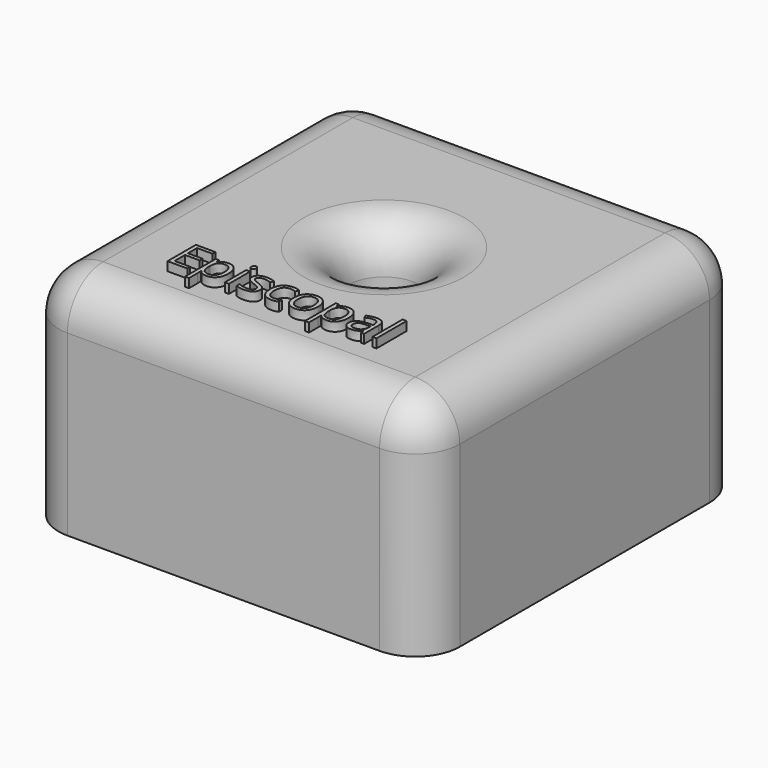
from build123d import *

# Parameters (mm, degrees)
F0_W         = 45
F0_H         = 45
F1_DEPTH     = 25
F2_R         = 4
F3_DEPTH     = 20
F4_R         = 5
F5_TEXT_SIZE = 5.5555555556
F6_DEPTH     = 1


# Not quite as in the source:
# - Text() gives the source's letters only with a copy of the font that has no kerning and outlines rounded to 1/6400 em; it was checked with that copy


with BuildPart() as f1:
    # F0 (on Top) → F1 (new body)
    with BuildSketch(Plane.XY):
        with Locations((-0.4572216421, 8.4124001385)):
            Rectangle(F0_W, F0_H)
    extrude(amount=F1_DEPTH)

    # F2 (on face) → F3 (cut)
    with BuildSketch(Plane.XY.offset(25)):
        with Locations((-0.4572216421, 8.4124001385)):
            Circle(F2_R)
    extrude(amount=-F3_DEPTH, mode=Mode.SUBTRACT)

    # F4
    f4_edges = [f1.edges().sort_by_distance(p)[0] for p in [
        (22.042778, 8.4124, 25),
        (-0.457222, -14.0876, 25),
        (-0.457222, 30.9124, 25),
        (-22.957222, 8.4124, 25),
        (-4.457222, 8.4124, 25),
        (-22.957222, 30.9124, 12.5),
        (22.042778, 30.9124, 12.5),
        (22.042778, -14.0876, 12.5),
        (-22.957222, -14.0876, 12.5),
    ]]
    fillet(f4_edges, radius=F4_R)

    # F5 (on face) → F6 (join)
    with BuildSketch(Plane.XY.offset(25)):
        with Locations((-12.9680234164, -6.9705045358)):
            Text('Episcopal', F5_TEXT_SIZE, font='Open Sans', text_align=(TextAlign.LEFT, TextAlign.BOTTOM))
    extrude(amount=F6_DEPTH)


solid = f1.part
